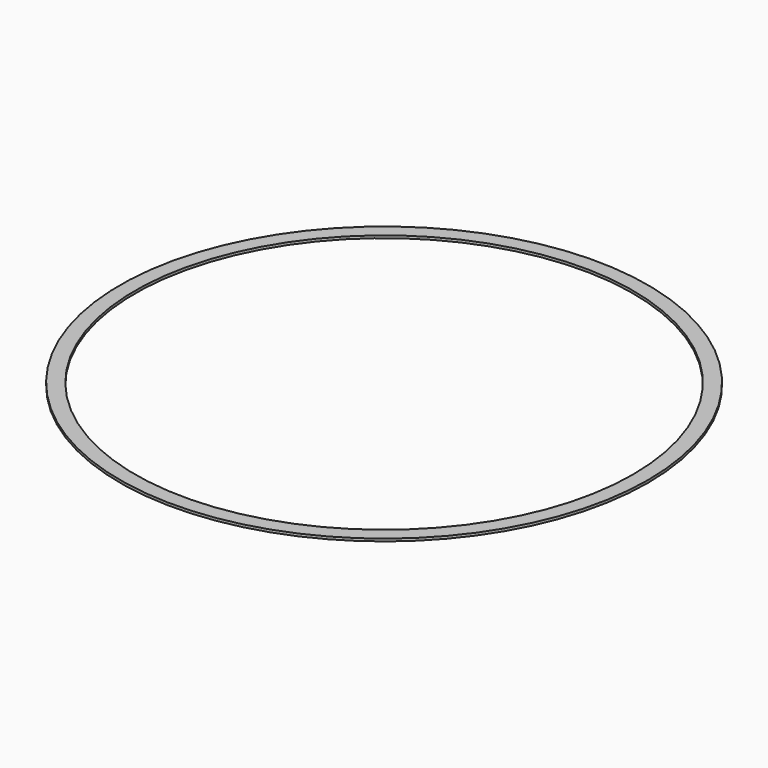
from build123d import *

# Parameters (mm, degrees)
F0_R     = 446.73139
F0_R_2   = 421.33139
F1_DEPTH = 4.2333333333


# Not quite as in the source:
# - a length typed as a fraction of an inch, garbled in the dataset ("3 / 203.2 mm" for 3/8 in), is restored


with BuildPart() as f1:
    # F0 (on Top) → F1 (new body)
    with BuildSketch(Plane.XY):
        Circle(F0_R)
        Circle(F0_R_2, mode=Mode.SUBTRACT)
    extrude(amount=F1_DEPTH)


solid = f1.part
